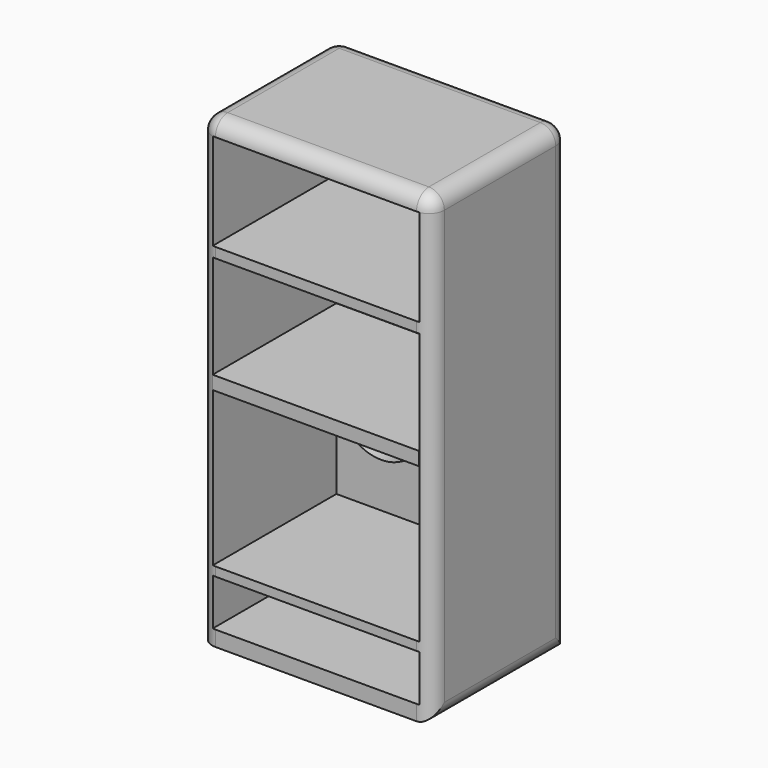
from build123d import *

# Parameters (mm, degrees)
F0_W         = 76.2
F0_H         = 152.4
F0_W_2       = 67.8425729275
F0_H_2       = 3.318388015
F0_H_3       = 2.9496736825
F1_DEPTH     = 50.8
F2_W         = 76.2
F2_H         = 152.4
F2_W_2       = 67.8425729275
F2_H_2       = 15.301451087
F2_H_3       = 89.0433862805
F2_H_4       = 31.7090302706
F3_DEPTH     = 5.08
F4_T1_DEPTH  = 81.28
F4_T3_DEPTH  = 177.8
F5_T1_DEPTH  = 66.04
F5_S5_W      = 5.08
F5_S5_H      = 5.08
F5_T6_DEPTH  = 5.08
F5_S11_W     = 5.08
F5_S11_H     = 5.08
F5_T12_DEPTH = 5.08
F6_T1_DEPTH  = 160.02
F6_T3_DEPTH  = 66.04
F6_S7_W      = 5.08
F6_S7_H      = 5.08
F6_T8_DEPTH  = 5.08
F6_T12_ANGLE = 89.9999999979
F7_W         = 67.8425729275
F7_H         = 4.4245161116
F8_DEPTH     = 50.8
F9_R         = 14.2326914524
F10_DEPTH    = 25.4


# Not quite as in the source:
# - a fillet or chamfer that OpenCascade refuses, or shapes differently, is made with other operations: its cross-section is extruded or revolved along the edge and cut away or added


with BuildPart() as f1:
    # F0 (on Front) → F1 (new body)
    with BuildSketch(Plane.XZ):
        Rectangle(F0_W, F0_H)
        Polygon((-33.9212864637, 71.1609646678), (33.9212864637, 71.1609646678), (33.9212864637, 39.4519343972), (33.9212864637, 36.1335463822), (33.9212864637, -52.9098398983), (33.9212864637, -55.8595135808), (33.9212864637, -71.1609646678), (-33.9212864637, -71.1609646678), (-33.9212864637, -55.8595135808), (-33.9212864637, -52.9098398983), (-33.9212864637, 36.1335463822), (-33.9212864637, 39.4519343972), align=None, mode=Mode.SUBTRACT)
        with Locations((0, 37.7927403897)):
            Rectangle(F0_W_2, F0_H_2)
        with Locations((0, -54.3846767396)):
            Rectangle(F0_W_2, F0_H_3)
    extrude(amount=F1_DEPTH)

    # F2 (on face) → F3 (join)
    with BuildSketch(Plane(origin=(0, 0, 0), x_dir=(-1, 0, 0), z_dir=(0, 1, 0))):
        Rectangle(F2_W, F2_H)
        with Locations((0, -63.5102391243)):
            Rectangle(F2_W_2, F2_H_2, mode=Mode.SUBTRACT)
        with Locations((0, -8.3881467581)):
            Rectangle(F2_W_2, F2_H_3, mode=Mode.SUBTRACT)
        with Locations((0, 55.3064495325)):
            Rectangle(F2_W_2, F2_H_4, mode=Mode.SUBTRACT)
        with Locations((0, 55.3064495325)):
            Rectangle(F2_W_2, F2_H_4)
        with Locations((0, -63.5102391243)):
            Rectangle(F2_W_2, F2_H_2)
        with Locations((0, -8.3881467581)):
            Rectangle(F2_W_2, F2_H_3)
    extrude(amount=F3_DEPTH)

    # F4: fillet of radius 5.08 on 6 edges, made by hand

    # F4_s2 → F4_t1 (cut)
    with BuildSketch(Plane.XZ.offset(-17.78)):
        with BuildLine():
            ThreePointArc((38.1, -71.12), (36.6121024484, -74.7121024484), (33.02, -76.2))
            Line((33.02, -76.2), (38.1, -76.2))
            Line((38.1, -76.2), (38.1, -71.12))
        make_face()
        with BuildLine():
            ThreePointArc((38.1, 71.12), (36.6121024484, 74.7121024484), (33.02, 76.2))
            Line((33.02, 76.2), (38.1, 76.2))
            Line((38.1, 76.2), (38.1, 71.12))
        make_face()
        with BuildLine():
            ThreePointArc((-38.1, 71.12), (-36.6121024484, 74.7121024484), (-33.02, 76.2))
            Line((-33.02, 76.2), (-38.1, 76.2))
            Line((-38.1, 76.2), (-38.1, 71.12))
        make_face()
    extrude(amount=F4_T1_DEPTH, mode=Mode.SUBTRACT)

    # F4_s4 → F4_t3 (cut)
    with BuildSketch(Plane.XY.offset(-88.9)):
        with BuildLine():
            ThreePointArc((38.1, -45.72), (36.6121024484, -49.3121024484), (33.02, -50.8))
            Line((33.02, -50.8), (38.1, -50.8))
            Line((38.1, -50.8), (38.1, -45.72))
        make_face()
        with BuildLine():
            ThreePointArc((38.1, 0), (36.6121024484, 3.5921024484), (33.02, 5.08))
            Line((33.02, 5.08), (38.1, 5.08))
            Line((38.1, 5.08), (38.1, 0))
        make_face()
        with BuildLine():
            ThreePointArc((-33.02, 5.08), (-36.6121024484, 3.5921024484), (-38.1, 0))
            Line((-38.1, 0), (-38.1, 5.08))
            Line((-38.1, 5.08), (-33.02, 5.08))
        make_face()
    extrude(amount=F4_T3_DEPTH, mode=Mode.SUBTRACT)

    # F5: fillet of radius 5.08 on 1 edges, made by hand

    # F5_s2 → F5_t1 (cut)
    with BuildSketch(Plane.YZ.offset(-33.02)):
        with BuildLine():
            ThreePointArc((5.08, 71.12), (3.5921024484, 74.7121024484), (0, 76.2))
            Line((0, 76.2), (5.08, 76.2))
            Line((5.08, 76.2), (5.08, 71.12))
        make_face()
    extrude(amount=F5_T1_DEPTH, mode=Mode.SUBTRACT)


with BuildPart() as f5_tool4:
    # F5_s5 → F5_t6 (new body)
    with BuildSketch(Plane.XZ):
        with Locations((-35.56, 73.66)):
            Rectangle(F5_S5_W, F5_S5_H)
    extrude(amount=-F5_T6_DEPTH)

    # F5_s7 → F5_t8 (revolve, cut)
    with BuildSketch(Plane(origin=(-33.02, 0, 71.12), x_dir=(0.7071067812, 0, -0.7071067812), z_dir=(0.7071067812, 0, 0.7071067812))):
        with BuildLine():
            ThreePointArc((0, -5.08), (5.08, 0), (0, 5.08))
            Line((0, 5.08), (0, -5.08))
        make_face()
    revolve(axis=Axis((-33.02, 0, 71.12), (0, 1, 0)), mode=Mode.SUBTRACT)


with BuildPart() as f1_1:
    add(f1.part)

    # F5_t3: cut F5_tool4
    add(f5_tool4.part, mode=Mode.SUBTRACT)


with BuildPart() as f5_tool10:
    # F5_s11 → F5_t12 (new body)
    with BuildSketch(Plane.XZ):
        with Locations((35.56, 73.66)):
            Rectangle(F5_S11_W, F5_S11_H)
    extrude(amount=-F5_T12_DEPTH)

    # F5_s13 → F5_t14 (revolve, cut)
    with BuildSketch(Plane(origin=(33.02, 0, 71.12), x_dir=(-0.7071067812, 0, -0.7071067812), z_dir=(0.7071067812, 0, -0.7071067812))):
        with BuildLine():
            ThreePointArc((0, -5.08), (5.08, 0), (0, 5.08))
            Line((0, 5.08), (0, -5.08))
        make_face()
    revolve(axis=Axis((33.02, 0, 71.12), (0, 1, 0)), mode=Mode.SUBTRACT)


with BuildPart() as f1_2:
    add(f1_1.part)

    # F5_t9: cut F5_tool10
    add(f5_tool10.part, mode=Mode.SUBTRACT)

    # F6: fillet of radius 5.08 on 1 edges, made by hand

    # F6_s2 → F6_t1 (cut)
    with BuildSketch(Plane.XY.offset(-88.9)):
        with BuildLine():
            ThreePointArc((-33.02, -50.8), (-36.6121024484, -49.3121024484), (-38.1, -45.72))
            Line((-38.1, -45.72), (-38.1, -50.8))
            Line((-38.1, -50.8), (-33.02, -50.8))
        make_face()
    extrude(amount=F6_T1_DEPTH, mode=Mode.SUBTRACT)

    # F6_s4 → F6_t3 (cut)
    with BuildSketch(Plane.YZ.offset(-33.02)):
        with BuildLine():
            ThreePointArc((-45.72, 76.2), (-49.3121024484, 74.7121024484), (-50.8, 71.12))
            Line((-50.8, 71.12), (-50.8, 76.2))
            Line((-50.8, 76.2), (-45.72, 76.2))
        make_face()
    extrude(amount=F6_T3_DEPTH, mode=Mode.SUBTRACT)


with BuildPart() as f6_tool6:
    # F6_s7 → F6_t8 (new body)
    with BuildSketch(Plane.XY.offset(71.12)):
        with Locations((35.56, -48.26)):
            Rectangle(F6_S7_W, F6_S7_H)
    extrude(amount=F6_T8_DEPTH)

    # F6_s9 → F6_t10 (revolve, cut)
    with BuildSketch(Plane(origin=(33.02, -45.72, 71.12), x_dir=(-0.7071067812, 0.7071067812, 0), z_dir=(0.7071067812, 0.7071067812, 0))):
        with BuildLine():
            ThreePointArc((0, -5.08), (5.08, 0), (0, 5.08))
            Line((0, 5.08), (0, -5.08))
        make_face()
    revolve(axis=Axis((33.02, -45.72, 71.12), (0, 0, 1)), mode=Mode.SUBTRACT)


with BuildPart() as f1_3:
    add(f1_2.part)

    # F6_t5: cut F6_tool6
    add(f6_tool6.part, mode=Mode.SUBTRACT)

    # F6_s11 → F6_t12 (revolve, cut)
    with BuildSketch(Plane.XY.offset(71.1199999999)):
        with BuildLine():
            ThreePointArc((-33.02, -50.8), (-36.6121024484, -49.3121024484), (-38.1, -45.72))
            Line((-38.1, -45.72), (-38.1, -50.8))
            Line((-38.1, -50.8), (-33.02, -50.8))
        make_face()
    revolve(axis=Axis((-33.0199999999, -50.8, 71.1199999999), (0, 1, 0)), revolution_arc=F6_T12_ANGLE, mode=Mode.SUBTRACT)

    # F7 (on face) → F8 (join)
    with BuildSketch(Plane.XZ):
        Rectangle(F7_W, F7_H)
    extrude(amount=F8_DEPTH)

    # F9 (on face) → F10 (cut)
    with BuildSketch(Plane(origin=(0, 5.08, 0), x_dir=(-1, 0, 0), z_dir=(0, 1, 0))):
        with Locations((19.2330349237, -24.0364484489)):
            Circle(F9_R)
    extrude(amount=-F10_DEPTH, mode=Mode.SUBTRACT)


solid = f1_3.part
